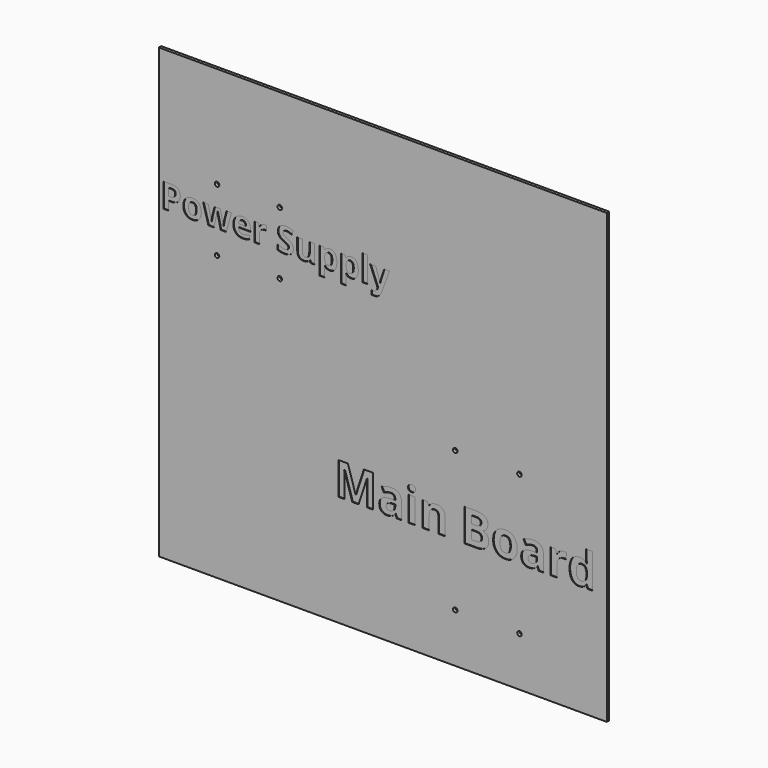
from build123d import *

# Parameters (mm, degrees)
F0_W           = 300
F0_H           = 300
F1_DEPTH       = 2
F2_R           = 1.5
F3_DEPTH       = 2
F4_R           = 1.5
F5_DEPTH       = 2
F6_TEXT_SIZE   = 22.6904379411
F6_TEXT_SIZE_2 = 30.4902748515
F7_DEPTH       = 0.5


# Not quite as in the source:
# - Text() gives the source's letters only with a copy of the font that has no kerning and outlines rounded to 1/6400 em; it was checked with that copy


with BuildPart() as f1:
    # F0 (on Front) → F1 (new body)
    with BuildSketch(Plane.XZ):
        Rectangle(F0_W, F0_H)
    extrude(amount=-F1_DEPTH)

    # F2 (on face) → F3 (cut, through all)
    with BuildSketch(Plane.XZ):
        with Locations((48.5, -23)):
            Circle(F2_R)
        with Locations((91.5, -23)):
            Circle(F2_R)
        with Locations((48.5, -117)):
            Circle(F2_R)
        with Locations((91.5, -117)):
            Circle(F2_R)
    extrude(amount=-F3_DEPTH, mode=Mode.SUBTRACT)

    # F4 (on face) → F5 (cut, through all)
    with BuildSketch(Plane.XZ):
        with Locations((-111, 82.0769896805)):
            Circle(F4_R)
        with Locations((-69, 82.0769896805)):
            Circle(F4_R)
        with Locations((-69, 40.0769896805)):
            Circle(F4_R)
        with Locations((-111, 40.0769896805)):
            Circle(F4_R)
    extrude(amount=-F5_DEPTH, mode=Mode.SUBTRACT)

    # F6 (on face) → F7 (cut)
    with BuildSketch(Plane.XZ):
        with Locations((-148.8209264353, 55.9035688639)):
            Text('Power Supply', F6_TEXT_SIZE, font='Open Sans', font_style=FontStyle.BOLD, text_align=(TextAlign.LEFT, TextAlign.BOTTOM))
        with Locations((-32.418963965, -75.8144259453)):
            Text('Main Board', F6_TEXT_SIZE_2, font='Open Sans', font_style=FontStyle.BOLD, text_align=(TextAlign.LEFT, TextAlign.BOTTOM))
    extrude(amount=-F7_DEPTH, mode=Mode.SUBTRACT)


solid = f1.part
